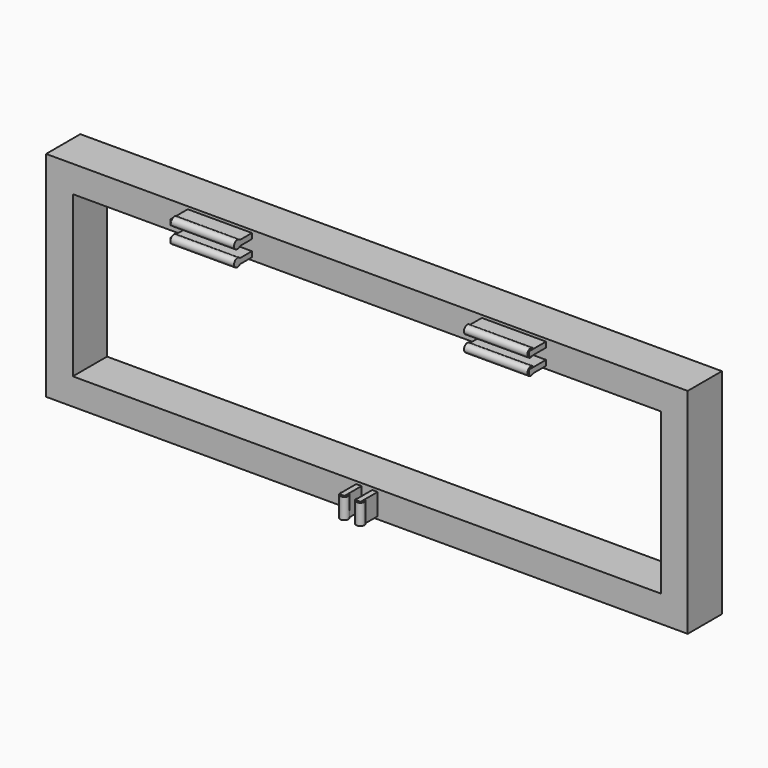
from build123d import *

# Parameters (mm, degrees)
F0_W      = 76.2
F0_H      = 25.4
F0_W_2    = 69.85
F0_H_2    = 19.05
F1_DEPTH  = 5.08
F2_W      = 7.62
F2_H      = 0.635
F3_DEPTH  = 1.778
F4_W      = 0.635
F4_H      = 2.54
F5_DEPTH  = 1.778
F6_W      = 0.1422071991
F6_H      = 0.635
F7_DEPTH  = 0.762
F8_R      = 0.4959508544
F9_DEPTH  = 7.4777928009
F10_W     = 0.0690778879
F10_H     = 0.635
F11_DEPTH = 0.762
F12_R     = 0.4959508544
F13_DEPTH = 7.5509221121
F14_W     = 0.095821996
F14_H     = 0.635
F15_DEPTH = 0.762
F16_R     = 0.4959508544
F17_DEPTH = 7.524178004
F18_W     = 0.0717212304
F18_H     = 0.635
F19_DEPTH = 0.762
F20_R     = 0.4959508544
F21_DEPTH = 7.5482787696
F22_W     = 0.635
F22_H     = 0.1154780363
F23_DEPTH = 0.762
F24_R     = 0.4959508544
F25_DEPTH = 2.4245219637
F26_W     = 0.635
F26_H     = 0.1073694763
F27_DEPTH = 0.762
F28_R     = 0.4959508544
F29_DEPTH = 2.4326305237


with BuildPart() as f1:
    # F0 (on Front) → F1 (new body)
    with BuildSketch(Plane.XZ):
        with Locations((8.76239234, 5.4013291374)):
            Rectangle(F0_W, F0_H)
        with Locations((8.76239234, 5.4013291374)):
            Rectangle(F0_W_2, F0_H_2, mode=Mode.SUBTRACT)
    extrude(amount=F1_DEPTH)

    # F2 (on face) → F3 (join)
    with BuildSketch(Plane.XZ.offset(5.08)):
        with Locations((26.22489234, 17.4663291374)):
            Rectangle(F2_W, F2_H)
        with Locations((26.22489234, 15.5613291374)):
            Rectangle(F2_W, F2_H)
        with Locations((-8.70010766, 17.4663291374)):
            Rectangle(F2_W, F2_H)
        with Locations((-8.70010766, 15.5613291374)):
            Rectangle(F2_W, F2_H)
    extrude(amount=F3_DEPTH)

    # F4 (on face) → F5 (join)
    with BuildSketch(Plane.XZ.offset(5.08)):
        with Locations((9.71489234, -5.7111708626)):
            Rectangle(F4_W, F4_H)
        with Locations((7.80989234, -5.7111708626)):
            Rectangle(F4_W, F4_H)
    extrude(amount=F5_DEPTH)

    # F6 (on face) → F7 (join)
    with BuildSketch(Plane.XZ.offset(6.858)):
        with Locations((-12.4390040605, 17.4663291374)):
            Rectangle(F6_W, F6_H)
    extrude(amount=F7_DEPTH)

    # F8 (on face) → F9 (join, through all)
    with BuildSketch(Plane.YZ.offset(-12.367900461)):
        with Locations((-7.239, 17.4663291374)):
            Circle(F8_R)
    extrude(amount=F9_DEPTH)

    # F10 (on face) → F11 (join)
    with BuildSketch(Plane.XZ.offset(6.858)):
        with Locations((-12.4755687161, 15.5613291374)):
            Rectangle(F10_W, F10_H)
    extrude(amount=F11_DEPTH)

    # F12 (on face) → F13 (join, through all)
    with BuildSketch(Plane.YZ.offset(-12.4410297722)):
        with Locations((-7.239, 15.5613291374)):
            Circle(F12_R)
    extrude(amount=F13_DEPTH)

    # F14 (on face) → F15 (join)
    with BuildSketch(Plane.XZ.offset(6.858)):
        with Locations((29.986981342, 17.4663291374)):
            Rectangle(F14_W, F14_H)
    extrude(amount=F15_DEPTH)

    # F16 (on face) → F17 (join, through all)
    with BuildSketch(Plane(origin=(29.939070344, 0, 0), x_dir=(0, -1, 0), z_dir=(-1, 0, 0))):
        with Locations((7.239, 17.4663291374)):
            Circle(F16_R)
    extrude(amount=F17_DEPTH)

    # F18 (on face) → F19 (join)
    with BuildSketch(Plane.XZ.offset(6.858)):
        with Locations((29.9990317248, 15.5613291374)):
            Rectangle(F18_W, F18_H)
    extrude(amount=F19_DEPTH)

    # F20 (on face) → F21 (join, through all)
    with BuildSketch(Plane(origin=(29.9631711096, 0, 0), x_dir=(0, -1, 0), z_dir=(-1, 0, 0))):
        with Locations((7.239, 15.5613291374)):
            Circle(F20_R)
    extrude(amount=F21_DEPTH)

    # F22 (on face) → F23 (join)
    with BuildSketch(Plane.XZ.offset(6.858)):
        with Locations((7.80989234, -4.4989098807)):
            Rectangle(F22_W, F22_H)
    extrude(amount=F23_DEPTH)

    # F24 (on face) → F25 (join, through all)
    with BuildSketch(Plane(origin=(0, 0, -4.5566488989), x_dir=(1, 0, 0), z_dir=(0, 0, -1))):
        with Locations((7.80989234, 7.239)):
            Circle(F24_R)
    extrude(amount=F25_DEPTH)

    # F26 (on face) → F27 (join)
    with BuildSketch(Plane.XZ.offset(6.858)):
        with Locations((9.71489234, -4.4948556007)):
            Rectangle(F26_W, F26_H)
    extrude(amount=F27_DEPTH)

    # F28 (on face) → F29 (join, through all)
    with BuildSketch(Plane(origin=(0, 0, -4.5485403389), x_dir=(1, 0, 0), z_dir=(0, 0, -1))):
        with Locations((9.71489234, 7.239)):
            Circle(F28_R)
    extrude(amount=F29_DEPTH)


solid = f1.part
